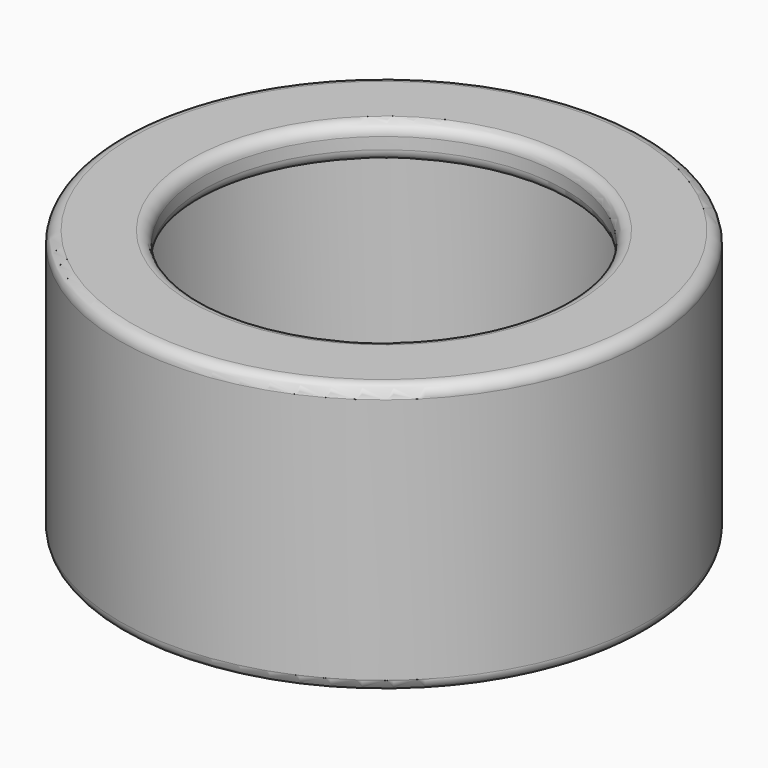
from build123d import *


with BuildPart() as f1:
    # F0 (on Right) → F1 (revolve)
    with BuildSketch(Plane.YZ):
        with BuildLine():
            Line((21.45, 3), (16.45, 3))
            ThreePointArc((16.45, 3), (15.7428932188, 2.7071067812), (15.45, 2))
            Line((15.45, 2), (15.45, 1))
            ThreePointArc((15.45, 1), (15.7428932188, 0.2928932188), (16.45, 0))
            Line((16.45, 0), (17.45, 0))
            Line((17.45, 0), (17.45, -19))
            ThreePointArc((17.45, -19), (17.7428932188, -19.7071067812), (18.45, -20))
            Line((18.45, -20), (21.45, -20))
            ThreePointArc((21.45, -20), (22.1571067812, -19.7071067812), (22.45, -19))
            Line((22.45, -19), (22.45, 2))
            ThreePointArc((22.45, 2), (22.1571067812, 2.7071067812), (21.45, 3))
        make_face()
    revolve(axis=Axis((0, 0, -3.255167976), (0, 0, -1)))


solid = f1.part
